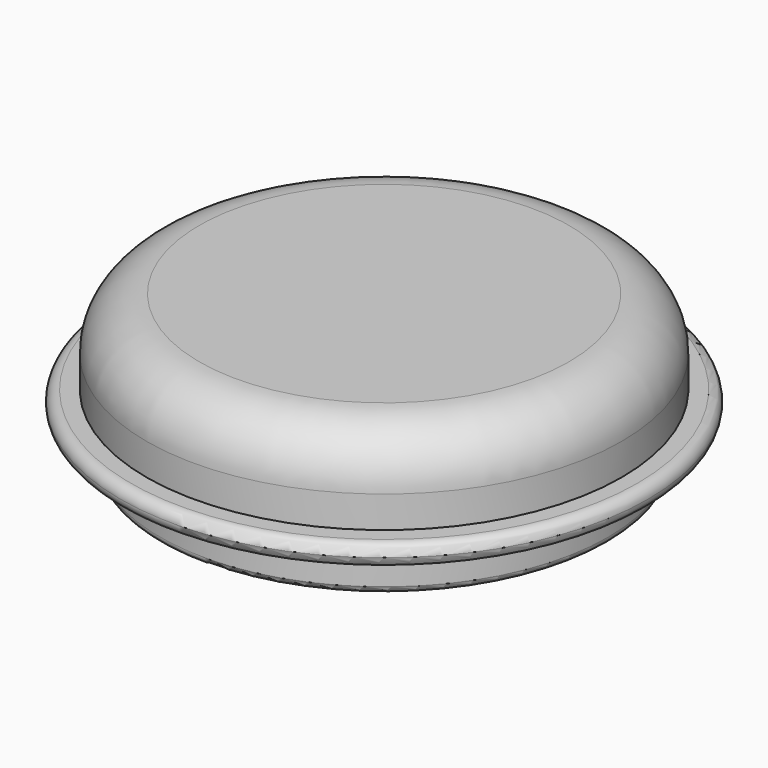
from build123d import *

# Parameters (mm, degrees)
F0_R          = 45
F0_R_2        = 42.5
F1_DEPTH      = 20
F0_R_3        = 50
F2_DEPTH      = 4
F3_R          = 42.5
F4_DEPTH      = 3.5
F0_R_4        = 40
F5_DEPTH      = 2
F5_DEPTH_BACK = 8
F6_R          = 10
F7_R          = 1.99999
F8_R          = 1.24999


# Not quite as in the source:
# - a fillet or chamfer is up to 0.001 mm smaller than in the source, because OpenCascade refuses the exact size


with BuildPart() as f1:
    # F0 (on Top) → F1 (new body)
    with BuildSketch(Plane.XY):
        Circle(F0_R)
        Circle(F0_R_2, mode=Mode.SUBTRACT)
    extrude(amount=F1_DEPTH)

    # F0 (on Top) → F2 (join)
    with BuildSketch(Plane.XY):
        Circle(F0_R_3)
        Circle(F0_R, mode=Mode.SUBTRACT)
    extrude(amount=F2_DEPTH)

    # F3 (on face) → F4 (join)
    with BuildSketch(Plane.XY.offset(20)):
        Circle(F3_R)
    extrude(amount=-F4_DEPTH)

    # F0 (on Top) → F5 (join, two sides)
    with BuildSketch(Plane.XY) as f5_sk:
        Circle(F0_R_2)
        Circle(F0_R_4, mode=Mode.SUBTRACT)
    extrude(amount=F5_DEPTH)
    extrude(f5_sk.sketch, amount=-F5_DEPTH_BACK)

    # F6
    f6_edges = [f1.edges().sort_by_distance(p)[0] for p in [
        (-42.5, 0, 16.5),
        (-45, 0, 20),
    ]]
    fillet(f6_edges, radius=F6_R)

    # F7 (radius 2 in the source; OpenCascade refuses exactly that, so slightly less here)
    f7_edges = [f1.edges().sort_by_distance(p)[0] for p in [
        (50, 0, 2),
        (-50, 0, 0),
        (-50, 0, 4),
    ]]
    fillet(f7_edges, radius=F7_R)

    # F8 (radius 1.25 in the source; OpenCascade refuses exactly that, so slightly less here)
    f8_edges = [f1.edges().sort_by_distance(p)[0] for p in [
        (-42.5, 0, -8),
        (-40, 0, -8),
        (42.5, 0, -4),
        (-42.5, 0, 0),
    ]]
    fillet(f8_edges, radius=F8_R)


solid = f1.part
